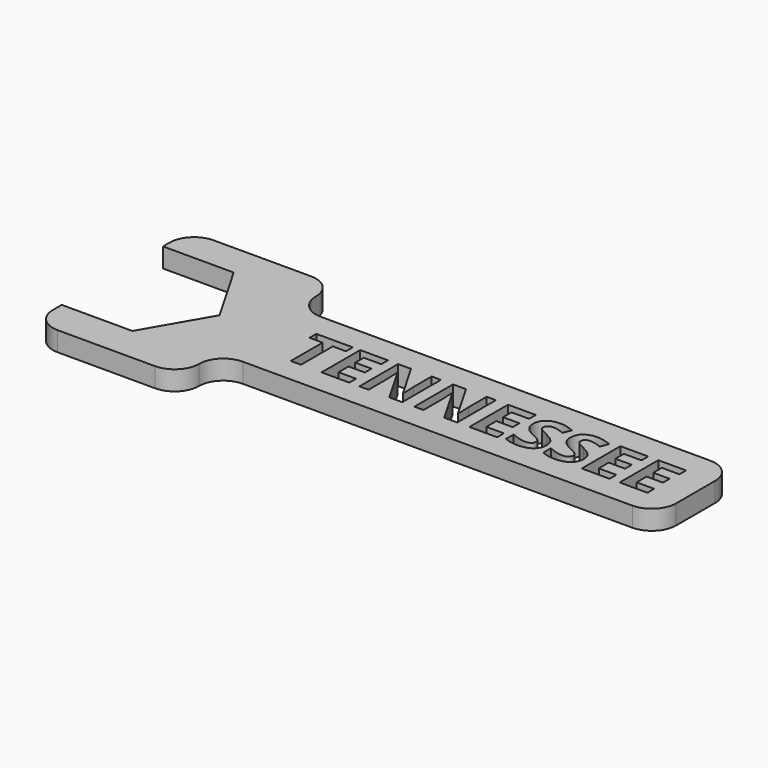
from build123d import *

# Parameters (mm, degrees)
F0_W         = 152.4
F0_H         = 50.8
F1_DEPTH     = 5.08
F3_DEPTH     = 5.081
F4_W         = 114.3
F4_H         = 12.7
F5_DEPTH     = 5.081
F6_R         = 6.34999
F7_TEXT_SIZE = 17.6388888889
F8_DEPTH     = 5.081


# Not quite as in the source:
# - a fillet or chamfer is up to 0.001 mm smaller than in the source, because OpenCascade refuses the exact size
# - Text() gives the source's letters only with a copy of the font that has no kerning and outlines rounded to 1/6400 em; it was checked with that copy


with BuildPart() as f1:
    # F0 (on Top) → F1 (new body)
    with BuildSketch(Plane.XY):
        with Locations((76.2, 25.4)):
            Rectangle(F0_W, F0_H)
    extrude(amount=F1_DEPTH)

    # F2 (on face) → F3 (cut, through all)
    with BuildSketch(Plane.XY.offset(5.08)):
        Polygon((27.9541058886, 25.7466956973), (18.4220529443, 42.2566956973), (0, 42.2566956973), (0, 9.2366956973), (18.4220529443, 9.2366956973), align=None)
    extrude(amount=-F3_DEPTH, mode=Mode.SUBTRACT)

    # F4 (on face) → F5 (cut, through all)
    with BuildSketch(Plane.XY.offset(5.08)):
        with Locations((95.25, 44.45)):
            Rectangle(F4_W, F4_H)
        with Locations((95.25, 6.35)):
            Rectangle(F4_W, F4_H)
    extrude(amount=-F5_DEPTH, mode=Mode.SUBTRACT)

    # F6 (radius 6.35 in the source; OpenCascade refuses exactly that, so slightly less here)
    f6_edges = [f1.edges().sort_by_distance(p)[0] for p in [
        (38.1, 0, 2.54),
        (152.4, 12.7, 2.54),
        (152.4, 38.1, 2.54),
        (38.1, 38.1, 2.54),
        (0, 50.8, 2.54),
        (0, 0, 2.54),
        (38.1, 12.7, 2.54),
        (38.1, 50.8, 2.54),
    ]]
    fillet(f6_edges, radius=F6_R)

    # F7 (on face) → F8 (cut, through all)
    with BuildSketch(Plane.XY.offset(5.08)):
        with Locations((48.1128255208, 19.05)):
            Text('TENNESSEE', F7_TEXT_SIZE, font='Open Sans', font_style=FontStyle.BOLD, text_align=(TextAlign.LEFT, TextAlign.BOTTOM))
    extrude(amount=-F8_DEPTH, mode=Mode.SUBTRACT)


solid = f1.part
